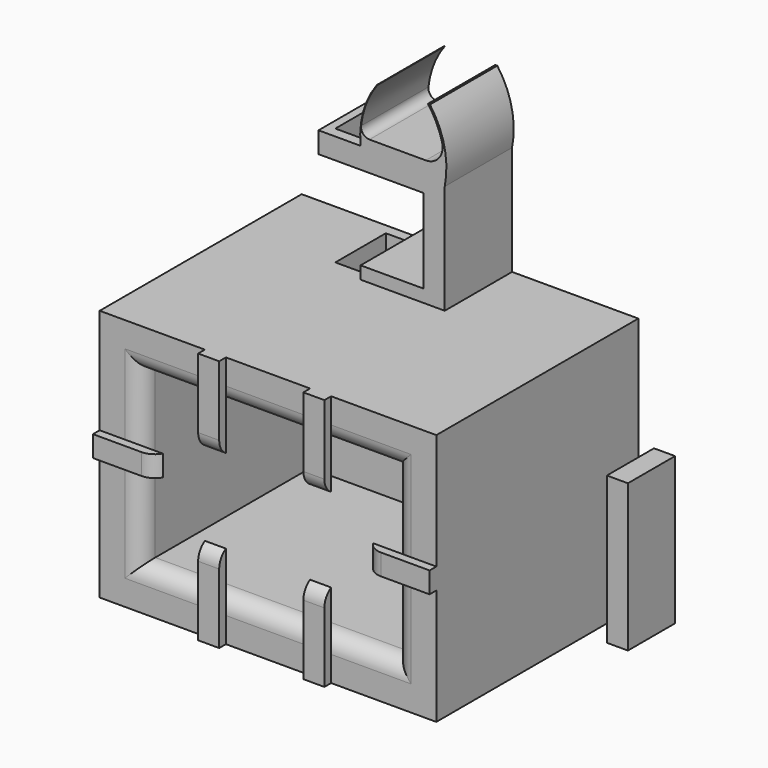
from build123d import *

# Parameters (mm, degrees)
F0_W        = 101.6
F0_H        = 76.2
F1_DEPTH    = 76.2
F2_T        = -12.7
F3_R        = 5.08
F4_W        = 6.35
F4_H        = 25.4
F4_W_2      = 19.05
F4_H_2      = 6.35
F5_DEPTH    = 2.54
F6_T1_DEPTH = 28.3470452561
F6_T3_DEPTH = 28.3470452561
F6_T5_DEPTH = 28.3470452561
F6_T7_DEPTH = 28.3470452561
F7_W        = 25.4
F7_H        = 38.1
F8_DEPTH    = 25.4
F9_W        = 25.4
F9_H        = 2.54
F10_ANGLE   = 45
F11_W       = 25.4
F11_H       = 5.08
F12_ANGLE   = 60
F13_START   = 15.24
F8_FACE2_W  = 25.4
F8_FACE2_H  = 25.4
F13_DEPTH   = 10.16
F14_R       = 2.54
F15_R       = 5.08
F16_W       = 25.4
F16_H       = 25.4
F17_DEPTH   = 19.05
F18_DEPTH   = 12.7
F20_DEPTH   = 44.45
F21_W       = 6.35
F21_H       = 17.78
F22_DEPTH   = 44.45


# Not quite as in the source:
# - a fillet or chamfer that OpenCascade refuses, or shapes differently, is made with other operations: its cross-section is extruded or revolved along the edge and cut away or added


with BuildPart() as f1:
    # F0 (on Front) → F1 (new body)
    with BuildSketch(Plane.XZ):
        with Locations((-50.8, 38.1)):
            Rectangle(F0_W, F0_H)
    extrude(amount=F1_DEPTH)

    # F2
    f2_openings = [f1.faces().sort_by_distance(p)[0] for p in [
        (-50.8, -76.2, 38.1),
    ]]
    offset(amount=F2_T, openings=f2_openings)

    # F3
    f3_edges = [f1.edges().sort_by_distance(p)[0] for p in [
        (-88.9, -76.2, 38.1),
        (-50.8, -76.2, 63.5),
        (-12.7, -76.2, 38.1),
        (-50.8, -76.2, 12.7),
    ]]
    fillet(f3_edges, radius=F3_R)

    # F4 (on face) → F5 (join)
    with BuildSketch(Plane.XZ.offset(76.2)):
        with Locations((-66.675, 63.5)):
            Rectangle(F4_W, F4_H)
        with Locations((-34.925, 63.5)):
            Rectangle(F4_W, F4_H)
        with Locations((-92.075, 41.275)):
            Rectangle(F4_W_2, F4_H_2)
        Polygon((0, 41.275), (-12.7, 41.275), (-19.05, 41.275), (-19.05, 34.925), (0, 34.925), align=None)
        with Locations((-66.675, 12.7)):
            Rectangle(F4_W, F4_H)
        with Locations((-34.925, 12.7)):
            Rectangle(F4_W, F4_H)
    extrude(amount=F5_DEPTH)

    # F6: fillet of radius 5.08 on 6 edges, made by hand

    # F6_s2 → F6_t1 (cut)
    with BuildSketch(Plane.XY.offset(27.1014773719)):
        with BuildLine():
            ThreePointArc((-82.55, -76.2), (-84.4094090512, -78.0594090512), (-86.9494090512, -78.74))
            Line((-86.9494090512, -78.74), (-82.55, -78.74))
            Line((-82.55, -78.74), (-82.55, -76.2))
        make_face()
    extrude(amount=F6_T1_DEPTH, mode=Mode.SUBTRACT)

    # F6_s4 → F6_t3 (cut)
    with BuildSketch(Plane.YZ.offset(-80.8485226281)):
        with BuildLine():
            ThreePointArc((-76.2, 50.8), (-78.0594090512, 52.6594090512), (-78.74, 55.1994090512))
            Line((-78.74, 55.1994090512), (-78.74, 50.8))
            Line((-78.74, 50.8), (-76.2, 50.8))
        make_face()
        with BuildLine():
            ThreePointArc((-76.2, 25.4), (-78.0594090512, 23.5405909488), (-78.74, 21.0005909488))
            Line((-78.74, 21.0005909488), (-78.74, 25.4))
            Line((-78.74, 25.4), (-76.2, 25.4))
        make_face()
    extrude(amount=F6_T3_DEPTH, mode=Mode.SUBTRACT)

    # F6_s6 → F6_t5 (cut)
    with BuildSketch(Plane.YZ.offset(-49.0985226281)):
        with BuildLine():
            ThreePointArc((-78.74, 55.1994090512), (-78.0594090512, 52.6594090512), (-76.2, 50.8))
            Line((-76.2, 50.8), (-78.74, 50.8))
            Line((-78.74, 50.8), (-78.74, 55.1994090512))
        make_face()
        with BuildLine():
            ThreePointArc((-76.2, 25.4), (-78.0594090512, 23.5405909488), (-78.74, 21.0005909488))
            Line((-78.74, 21.0005909488), (-78.74, 25.4))
            Line((-78.74, 25.4), (-76.2, 25.4))
        make_face()
    extrude(amount=F6_T5_DEPTH, mode=Mode.SUBTRACT)

    # F6_s8 → F6_t7 (cut)
    with BuildSketch(Plane.XY.offset(23.9264773719)):
        with BuildLine():
            ThreePointArc((-14.6505909488, -78.74), (-17.1905909488, -78.0594090512), (-19.05, -76.2))
            Line((-19.05, -76.2), (-19.05, -78.74))
            Line((-19.05, -78.74), (-14.6505909488, -78.74))
        make_face()
    extrude(amount=F6_T7_DEPTH, mode=Mode.SUBTRACT)

    # F7 (on face) → F8 (join)
    with BuildSketch(Plane(origin=(0, 0, 0), x_dir=(-1, 0, 0), z_dir=(0, 1, 0))):
        with Locations((50.8, 95.25)):
            Rectangle(F7_W, F7_H)
    extrude(amount=-F8_DEPTH)

    # F9 (on face) → F10 (revolve)
    with BuildSketch(Plane(origin=(-63.5, 0, 0), x_dir=(0, -1, 0), z_dir=(-1, 0, 0))):
        with Locations((12.7, 113.03)):
            Rectangle(F9_W, F9_H)
    revolve(axis=Axis((-38.1, -12.7, 114.3), (0, 1, 0)), revolution_arc=F10_ANGLE)

    # F11 (on face) → F12 (revolve)
    with BuildSketch(Plane.YZ.offset(-38.1)):
        with Locations((-12.7, 111.76)):
            Rectangle(F11_W, F11_H)
    revolve(axis=Axis((-63.5, -12.7, 114.3), (0, -1, 0)), revolution_arc=F12_ANGLE)

    # F8_face2 (on face) → F13 (cut)
    with BuildSketch(Plane(origin=(-50.8, -12.7, 114.3), x_dir=(1, 0, 0), z_dir=(0, 0, 1)).offset(F13_START)):
        Rectangle(F8_FACE2_W, F8_FACE2_H)
    extrude(amount=F13_DEPTH, mode=Mode.SUBTRACT)

    # F14
    f14_edges = [f1.edges().sort_by_distance(p)[0] for p in [
        (-63.5, -12.7, 114.3),
    ]]
    fillet(f14_edges, radius=F14_R)

    # F15
    f15_edges = [f1.edges().sort_by_distance(p)[0] for p in [
        (-38.1, -12.7, 114.3),
    ]]
    fillet(f15_edges, radius=F15_R)

    # F16 (on face) → F17 (cut)
    with BuildSketch(Plane(origin=(-63.5, 0, 0), x_dir=(0, -1, 0), z_dir=(-1, 0, 0))):
        with Locations((12.7, 92.71)):
            Rectangle(F16_W, F16_H)
    extrude(amount=-F17_DEPTH, mode=Mode.SUBTRACT)

    # F18 (add): a face of the model
    f18_faces = [f1.faces().sort_by_distance(p)[0] for p in [
        (-63.5, -12.7, 108.585),
    ]]
    extrude(f18_faces, amount=F18_DEPTH)

    # F19 (on face) → F20 (cut)
    with BuildSketch(Plane.XY.offset(111.76)):
        with BuildLine():
            ThreePointArc((-73.66, -12.7000000431), (-69.8499999784, -16.51), (-66.04, -12.7))
            ThreePointArc((-66.04, -12.7), (-69.8500000216, -8.89), (-73.66, -12.7000000431))
        make_face()
        with BuildLine():
            Line((-66.04, -22.225), (-66.04, -12.7))
            ThreePointArc((-66.04, -12.7), (-69.8499999784, -16.51), (-73.66, -12.7000000431))
            Line((-73.66, -12.7000000431), (-73.66, -22.225))
            Line((-73.66, -22.225), (-66.04, -22.225))
        make_face()
        with BuildLine():
            ThreePointArc((-73.66, -12.7000000431), (-69.8500000216, -8.89), (-66.04, -12.7))
            Line((-66.04, -12.7), (-66.04, -3.175))
            Line((-66.04, -3.175), (-73.66, -3.175))
            Line((-73.66, -3.175), (-73.66, -12.7000000431))
        make_face()
    extrude(amount=-F20_DEPTH, mode=Mode.SUBTRACT)


with BuildPart() as f22:
    # F21 (on Top) → F22 (new body)
    with BuildSketch(Plane.XY):
        with Locations((9.3328396462, -10.6671517172)):
            Rectangle(F21_W, F21_H)
    extrude(amount=F22_DEPTH)


solid = Compound([f1.part, f22.part])
